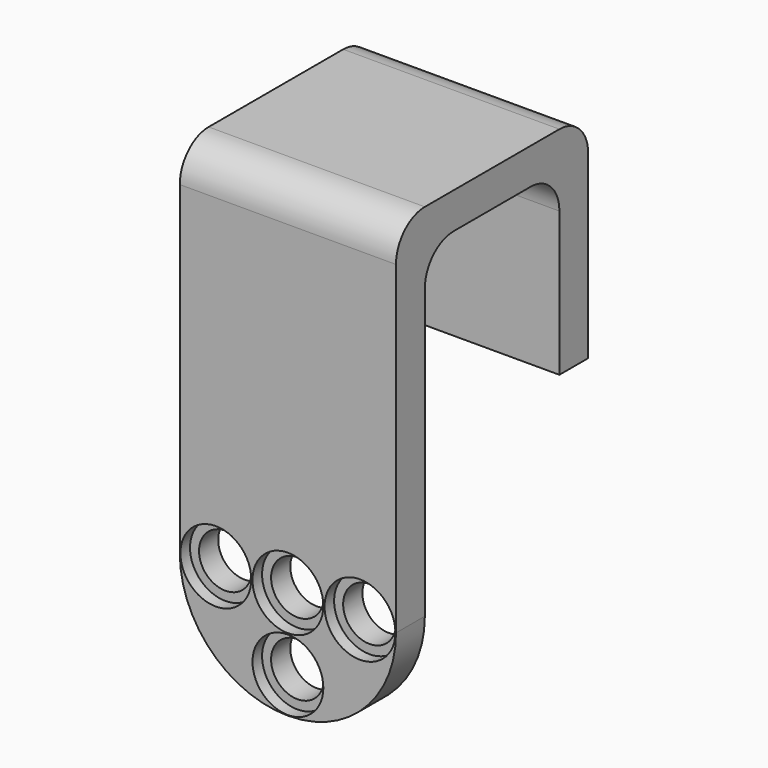
from build123d import *

# Parameters (mm, degrees)
F1_DEPTH = 18
F2_R     = 2.95
F2_R_2   = 2.2
F3_DEPTH = 1
F4_R     = 3
F5_R     = 2.2
F6_DEPTH = 20.001
F5_R_2   = 2.95
F7_DEPTH = 1


with BuildPart() as f1:
    # F0 (on Right) → F1 (new body)
    with BuildSketch(Plane.YZ):
        with BuildLine():
            Line((10, 0), (10, 15))
            ThreePointArc((10, 15), (9.1213203436, 17.1213203436), (7, 18))
            Line((7, 18), (-7, 18))
            ThreePointArc((-7, 18), (-9.1213203436, 17.1213203436), (-10, 15))
            Line((-10, 15), (-10, -21))
            Line((-10, -21), (-7, -21))
            Line((-7, -21), (-7, 15))
            Line((-7, 15), (7, 15))
            Line((7, 15), (7, 0))
            Line((7, 0), (10, 0))
        make_face()
    extrude(amount=F1_DEPTH)

    # F2 (on face) → F3 (cut)
    with BuildSketch(Plane(origin=(0, 10, 0), x_dir=(-1, 0, 0), z_dir=(0, 1, 0))):
        with Locations((-14.9964041635, 8.9979103986)):
            Circle(F2_R)
        with Locations((-14.9964041635, 8.9979103986)):
            Circle(F2_R_2, mode=Mode.SUBTRACT)
        with Locations((-8.9964041635, 8.9979103986)):
            Circle(F2_R)
        with Locations((-8.9964041635, 8.9979103986)):
            Circle(F2_R_2, mode=Mode.SUBTRACT)
        with Locations((-2.9964041635, 8.9979103986)):
            Circle(F2_R)
        with Locations((-2.9964041635, 8.9979103986)):
            Circle(F2_R_2, mode=Mode.SUBTRACT)
        with Locations((-8.9964041635, 2.9979103986)):
            Circle(F2_R)
        with Locations((-8.9964041635, 2.9979103986)):
            Circle(F2_R_2, mode=Mode.SUBTRACT)
    extrude(amount=-F3_DEPTH, mode=Mode.SUBTRACT)

    # F4
    f4_edges = [f1.edges().sort_by_distance(p)[0] for p in [
        (9, 7, 15),
        (9, -7, 15),
    ]]
    fillet(f4_edges, radius=F4_R)

    # F5 (on face) → F6 (cut, through all)
    with BuildSketch(Plane.XZ.offset(10)):
        with BuildLine():
            ThreePointArc((18, -12), (15.3639610307, -18.3639610307), (9, -21))
            Line((9, -21), (18, -21))
            Line((18, -21), (18, -12))
        make_face()
        with BuildLine():
            ThreePointArc((9, -21), (2.6360389693, -18.3639610307), (0, -12))
            Line((0, -12), (0, -21))
            Line((0, -21), (9, -21))
        make_face()
        with Locations((3, -12)):
            Circle(F5_R)
        with Locations((9, -12)):
            Circle(F5_R)
        with Locations((15, -12)):
            Circle(F5_R)
        with Locations((9, -18)):
            Circle(F5_R)
    extrude(amount=-F6_DEPTH, mode=Mode.SUBTRACT)

    # F5 (on face) → F7 (cut)
    with BuildSketch(Plane.XZ.offset(10)):
        with Locations((3, -12)):
            Circle(F5_R_2)
        with Locations((3, -12)):
            Circle(F5_R, mode=Mode.SUBTRACT)
        with Locations((9, -12)):
            Circle(F5_R_2)
        with Locations((9, -12)):
            Circle(F5_R, mode=Mode.SUBTRACT)
        with Locations((15, -12)):
            Circle(F5_R_2)
        with Locations((15, -12)):
            Circle(F5_R, mode=Mode.SUBTRACT)
        with Locations((9, -18)):
            Circle(F5_R_2)
        with Locations((9, -18)):
            Circle(F5_R, mode=Mode.SUBTRACT)
    extrude(amount=-F7_DEPTH, mode=Mode.SUBTRACT)


solid = f1.part
